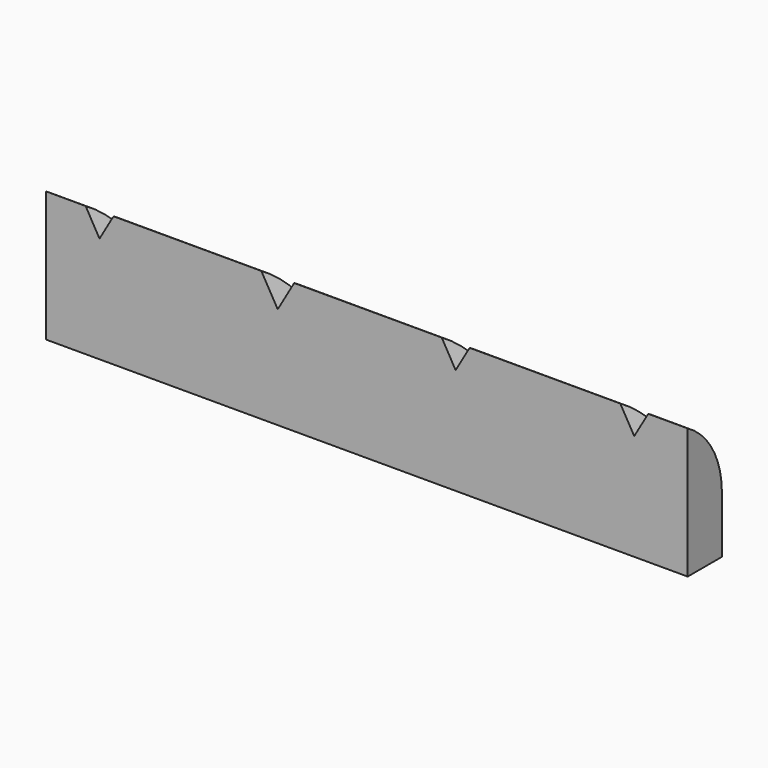
from build123d import *

# Parameters (mm, degrees)
F0_W        = 38.1
F0_H        = 2.54
F1_DEPTH    = 7.747
F3_T1_DEPTH = 60.0970452561
F4_DEPTH    = 25.4


# Not quite as in the source:
# - a fillet or chamfer that OpenCascade refuses, or shapes differently, is made with other operations: its cross-section is extruded or revolved along the edge and cut away or added


with BuildPart() as f1:
    # F0 (on Top) → F1 (new body)
    with BuildSketch(Plane.XY):
        with Locations((0, 1.27)):
            Rectangle(F0_W, F0_H)
    extrude(amount=F1_DEPTH)

    # F3: fillet of radius 5.08 on 1 edges, made by hand

    # F3_s2 → F3_t1 (cut)
    with BuildSketch(Plane.YZ.offset(-30.0485226281)):
        with BuildLine():
            ThreePointArc((2.54, 3.3475909488), (1.8594090512, 5.8875909488), (0, 7.747))
            Line((0, 7.747), (2.54, 7.747))
            Line((2.54, 7.747), (2.54, 3.3475909488))
        make_face()
    extrude(amount=F3_T1_DEPTH, mode=Mode.SUBTRACT)

    # F2 (on face) → F4 (cut)
    with BuildSketch(Plane.XZ):
        Polygon((-15.875, 6.3092954744), (-15.0449409051, 7.747), (-16.7050590949, 7.747), align=None)
        Polygon((-4.3191939367, 7.747), (-6.2726060633, 7.747), (-5.2959, 6.0552954744), align=None)
        Polygon((6.1005590949, 7.747), (4.4404409051, 7.747), (5.2705, 6.3092954744), align=None)
        Polygon((16.7050590949, 7.747), (15.0449409051, 7.747), (15.875, 6.3092954744), align=None)
    extrude(amount=-F4_DEPTH, mode=Mode.SUBTRACT)


solid = f1.part
